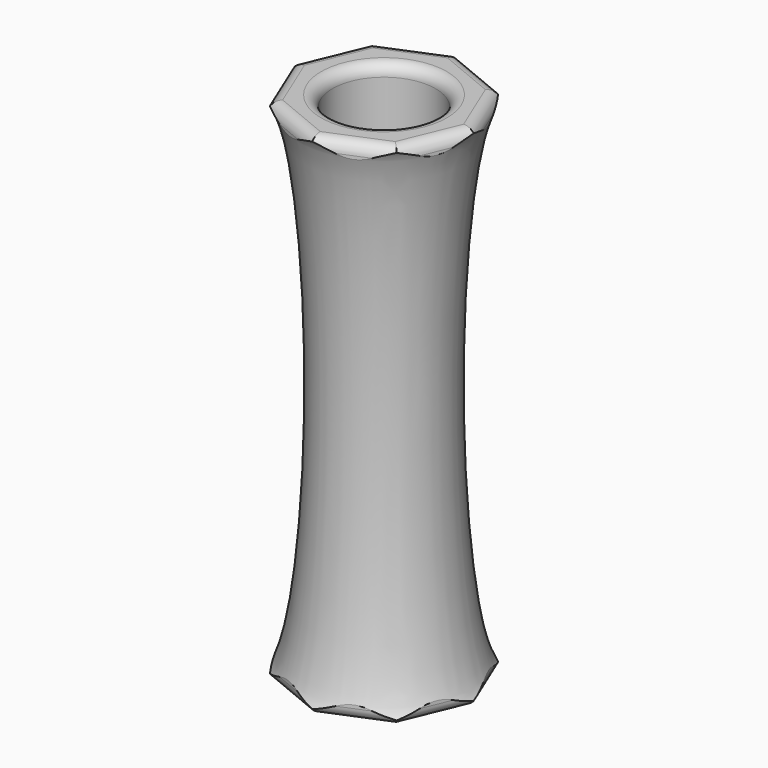
from build123d import *

# Parameters (mm, degrees)
F0_R         = 9.1
F1_DEPTH     = 90
F5_T1_DEPTH  = 22.4264068712
F5_T3_DEPTH  = 22.4264068712
F5_T5_DEPTH  = 22.4264068712
F5_T7_DEPTH  = 22.4264068712
F5_T9_DEPTH  = 22.4264068712
F5_T11_DEPTH = 22.4264068712
F5_T13_DEPTH = 22.4264068712
F5_T15_DEPTH = 22.4264068712


# Not quite as in the source:
# - a fillet or chamfer that OpenCascade refuses, or shapes differently, is made with other operations: its cross-section is extruded or revolved along the edge and cut away or added


with BuildPart() as f1:
    # F0 (on Top) → F1 (new body)
    with BuildSketch(Plane.XY):
        Polygon((16.2358830044, 0), (11.480502971, 11.480502971), (0, 16.2358830044), (-11.480502971, 11.480502971), (-16.2358830044, 0), (-11.480502971, -11.480502971), (0, -16.2358830044), (11.480502971, -11.480502971), align=None)
        Circle(F0_R, mode=Mode.SUBTRACT)
    extrude(amount=-F1_DEPTH)

    # F2 (on Front) → F4 (revolve, cut)
    with BuildSketch(Plane.XZ):
        with BuildLine():
            Line((25, 0), (17, 0))
            add(Edge.make_bspline(
                [(17, 0), (11, 0), (11, -45), (11, -90), (17, -90)],
                knots=[0, 0, 0, 1.5707963268, 1.5707963268, 3.1415926536, 3.1415926536, 3.1415926536], degree=2, weights=[1, 0.7071067812, 1, 0.7071067812, 1]))
            Line((17, -90), (25, -90))
            Line((25, -90), (25, 0))
        make_face()
    revolve(axis=Axis((0, 0, -44.5161331445), (0, 0, -1)), mode=Mode.SUBTRACT)

    # F5: fillet of radius 2 on 18 edges, made by hand

    # F5_s2 → F5_t1 (cut)
    with BuildSketch(Plane(origin=(-4.2911071785, -10.359649148, 0), x_dir=(0, 0, 1), z_dir=(0.3826834324, 0.9238795325, 0))):
        with BuildLine():
            ThreePointArc((-2, 15), (-0.5857864376, 14.4142135624), (0, 13))
            Line((0, 13), (0, 15))
            Line((0, 15), (-2, 15))
        make_face()
        with BuildLine():
            ThreePointArc((-88, 15), (-89.4142135624, 14.4142135624), (-90, 13))
            Line((-90, 13), (-90, 15))
            Line((-90, 15), (-88, 15))
        make_face()
    extrude(amount=F5_T1_DEPTH, mode=Mode.SUBTRACT)

    # F5_s4 → F5_t3 (cut)
    with BuildSketch(Plane(origin=(4.2911071785, -10.359649148, 0), x_dir=(0, 0, 1), z_dir=(-0.3826834324, 0.9238795325, 0))):
        with BuildLine():
            ThreePointArc((0, 13), (-0.5857864376, 14.4142135624), (-2, 15))
            Line((-2, 15), (0, 15))
            Line((0, 15), (0, 13))
        make_face()
        with BuildLine():
            ThreePointArc((-88, 15), (-89.4142135624, 14.4142135624), (-90, 13))
            Line((-90, 13), (-90, 15))
            Line((-90, 15), (-88, 15))
        make_face()
    extrude(amount=F5_T3_DEPTH, mode=Mode.SUBTRACT)

    # F5_s6 → F5_t5 (cut)
    with BuildSketch(Plane(origin=(10.359649148, -4.2911071785, 0), x_dir=(0, 0, 1), z_dir=(-0.9238795325, 0.3826834324, 0))):
        with BuildLine():
            ThreePointArc((0, 13), (-0.5857864376, 14.4142135624), (-2, 15))
            Line((-2, 15), (0, 15))
            Line((0, 15), (0, 13))
        make_face()
        with BuildLine():
            ThreePointArc((-88, 15), (-89.4142135624, 14.4142135624), (-90, 13))
            Line((-90, 13), (-90, 15))
            Line((-90, 15), (-88, 15))
        make_face()
    extrude(amount=F5_T5_DEPTH, mode=Mode.SUBTRACT)

    # F5_s8 → F5_t7 (cut)
    with BuildSketch(Plane(origin=(10.359649148, 4.2911071785, 0), x_dir=(0, 0, 1), z_dir=(-0.9238795325, -0.3826834324, 0))):
        with BuildLine():
            ThreePointArc((0, 13), (-0.5857864376, 14.4142135624), (-2, 15))
            Line((-2, 15), (0, 15))
            Line((0, 15), (0, 13))
        make_face()
        with BuildLine():
            ThreePointArc((-88, 15), (-89.4142135624, 14.4142135624), (-90, 13))
            Line((-90, 13), (-90, 15))
            Line((-90, 15), (-88, 15))
        make_face()
    extrude(amount=F5_T7_DEPTH, mode=Mode.SUBTRACT)

    # F5_s10 → F5_t9 (cut)
    with BuildSketch(Plane(origin=(4.2911071785, 10.359649148, 0), x_dir=(0, 0, 1), z_dir=(-0.3826834324, -0.9238795325, 0))):
        with BuildLine():
            ThreePointArc((0, 13), (-0.5857864376, 14.4142135624), (-2, 15))
            Line((-2, 15), (0, 15))
            Line((0, 15), (0, 13))
        make_face()
        with BuildLine():
            ThreePointArc((-88, 15), (-89.4142135624, 14.4142135624), (-90, 13))
            Line((-90, 13), (-90, 15))
            Line((-90, 15), (-88, 15))
        make_face()
    extrude(amount=F5_T9_DEPTH, mode=Mode.SUBTRACT)

    # F5_s12 → F5_t11 (cut)
    with BuildSketch(Plane(origin=(-4.2911071785, 10.359649148, 0), x_dir=(0, 0, 1), z_dir=(0.3826834324, -0.9238795325, 0))):
        with BuildLine():
            ThreePointArc((0, 13), (-0.5857864376, 14.4142135624), (-2, 15))
            Line((-2, 15), (0, 15))
            Line((0, 15), (0, 13))
        make_face()
        with BuildLine():
            ThreePointArc((-88, 15), (-89.4142135624, 14.4142135624), (-90, 13))
            Line((-90, 13), (-90, 15))
            Line((-90, 15), (-88, 15))
        make_face()
    extrude(amount=F5_T11_DEPTH, mode=Mode.SUBTRACT)

    # F5_s14 → F5_t13 (cut)
    with BuildSketch(Plane(origin=(-10.359649148, 4.2911071785, 0), x_dir=(0, 0, 1), z_dir=(0.9238795325, -0.3826834324, 0))):
        with BuildLine():
            ThreePointArc((0, 13), (-0.5857864376, 14.4142135624), (-2, 15))
            Line((-2, 15), (0, 15))
            Line((0, 15), (0, 13))
        make_face()
        with BuildLine():
            ThreePointArc((-88, 15), (-89.4142135624, 14.4142135624), (-90, 13))
            Line((-90, 13), (-90, 15))
            Line((-90, 15), (-88, 15))
        make_face()
    extrude(amount=F5_T13_DEPTH, mode=Mode.SUBTRACT)

    # F5_s16 → F5_t15 (cut)
    with BuildSketch(Plane(origin=(-10.359649148, -4.2911071785, 0), x_dir=(0, 0, 1), z_dir=(0.9238795325, 0.3826834324, 0))):
        with BuildLine():
            ThreePointArc((0, 13), (-0.5857864376, 14.4142135624), (-2, 15))
            Line((-2, 15), (0, 15))
            Line((0, 15), (0, 13))
        make_face()
        with BuildLine():
            ThreePointArc((-88, 15), (-89.4142135624, 14.4142135624), (-90, 13))
            Line((-90, 13), (-90, 15))
            Line((-90, 15), (-88, 15))
        make_face()
    extrude(amount=F5_T15_DEPTH, mode=Mode.SUBTRACT)

    # F5_s17 → F5_t18 (revolve, cut)
    with BuildSketch(Plane.XZ):
        with BuildLine():
            ThreePointArc((11.1, 0), (9.6857864376, -0.5857864376), (9.1, -2))
            Line((9.1, -2), (9.1, 0))
            Line((9.1, 0), (11.1, 0))
        make_face()
    revolve(axis=Axis((0, 0, 0), (0, 0, 1)), mode=Mode.SUBTRACT)

    # F5_s19 → F5_t20 (revolve, cut)
    with BuildSketch(Plane.XZ):
        with BuildLine():
            ThreePointArc((9.1, -88), (9.6857864376, -89.4142135624), (11.1, -90))
            Line((11.1, -90), (9.1, -90))
            Line((9.1, -90), (9.1, -88))
        make_face()
    revolve(axis=Axis((0, 0, -90), (0, 0, 1)), mode=Mode.SUBTRACT)


solid = f1.part
